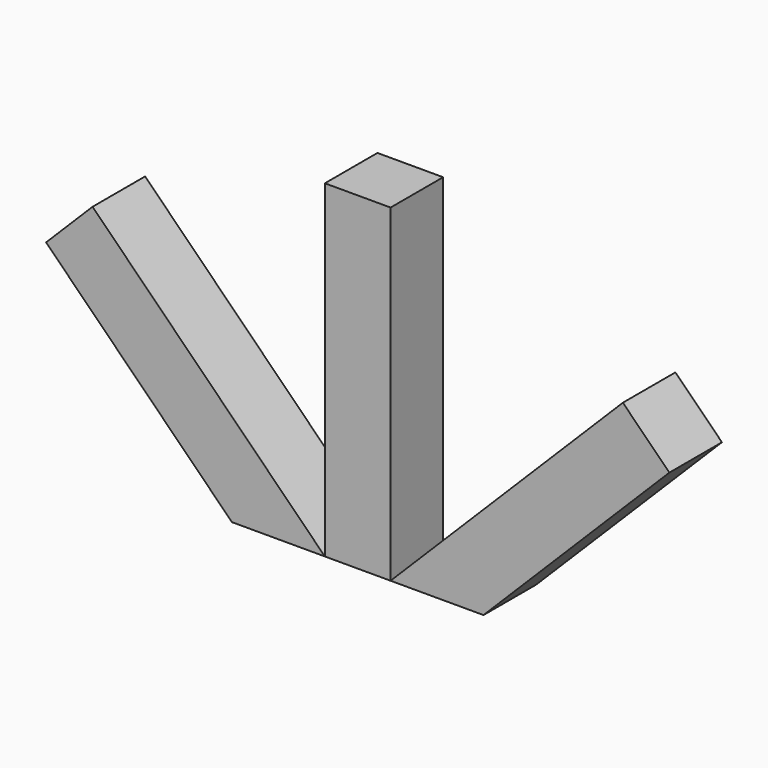
from build123d import *

# Parameters (mm, degrees)
F1_DEPTH = 10
F4_R     = 2
F6_DEPTH = 42.76


# Not quite as in the source:
# - the program builds the solid bodies; features that only make, move or delete a surface that nothing else refers to are left out


with BuildPart() as f1:
    # F0 (on Front) → F1 (new body)
    with BuildSketch(Plane.XZ):
        Polygon((40.3655851163, 10.3553390593), (5.010246057, -25), (19.1523816807, -25), (47.4366529281, 3.2842712475), align=None)
    extrude(amount=F1_DEPTH)

    # F4 (on face) → F6 (join)
    with BuildSketch(Plane(origin=(25.3604620878, 0, 25.3604620878), x_dir=(0.7071067812, 0, -0.7071067812), z_dir=(0.7071067812, 0, 0.7071067812))):
        with Locations((25.838650763, -5)):
            Circle(F4_R)
    extrude(amount=-F6_DEPTH)


with BuildPart() as f1b:
    # F0 (on Front) → F1, piece 2 (new body)
    with BuildSketch(Plane.XZ):
        Polygon((0.010246057, -25), (5.010246057, -25), (5.010246057, 25), (-4.989753943, 25), (-4.989753943, -25), align=None)
    extrude(amount=F1_DEPTH)


with BuildPart() as f1c:
    # F0 (on Front) → F1, piece 3 (new body)
    with BuildSketch(Plane.XZ):
        Polygon((-19.1318895668, -25), (-4.989753943, -25), (-40.3450930024, 10.3553390593), (-47.4161608142, 3.2842712475), align=None)
    extrude(amount=F1_DEPTH)


solid = Compound([f1.part, f1b.part, f1c.part])
